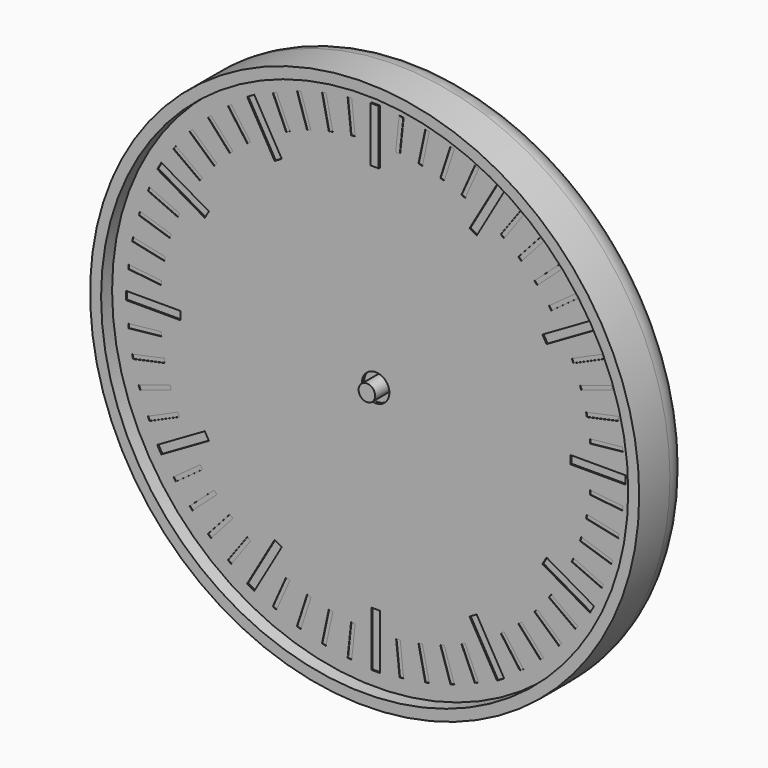
from build123d import *

# Parameters (mm, degrees)
F0_R      = 100
F1_DEPTH  = 24
F2_R      = 10
F3_T      = -4
F4_R      = 5
F4_R_2    = 3
F5_DEPTH  = 2
F6_DEPTH  = 19
F7_DEPTH  = 8
F9_DEPTH  = 4
F11_DEPTH = 4
F12_R     = 5
F12_R_2   = 3
F13_DEPTH = 2
F14_R     = 3
F15_DEPTH = 4
F17_DEPTH = 4
F18_R     = 3
F19_DEPTH = 2
F20_R     = 98
F20_R_2   = 5
F21_DEPTH = 1
F23_R     = 5
F23_R_2   = 3
F24_DEPTH = 2
F25_W     = 3
F25_H     = 20
F25_W_2   = 20
F25_H_2   = 3
F26_DEPTH = 0.5
F27_W     = 1.5
F27_H     = 12
F27_W_2   = 12
F27_H_2   = 1.5
F28_DEPTH = 0.2
F29_DEPTH = 1
F30_DEPTH = 0.4


with BuildPart() as f1:
    # F0 (on Front) → F1 (new body)
    with BuildSketch(Plane.XZ):
        Circle(F0_R)
    extrude(amount=F1_DEPTH)

    # F2
    f2_edges = [f1.edges().sort_by_distance(p)[0] for p in [
        (-100, 0, 0),
    ]]
    fillet(f2_edges, radius=F2_R)

    # F3
    f3_openings = [f1.faces().sort_by_distance(p)[0] for p in [
        (0, -24, 0),
    ]]
    offset(amount=F3_T, openings=f3_openings)

    # F4 (on face) → F5 (join)
    with BuildSketch(Plane.XZ.offset(4)):
        Circle(F4_R)
        Circle(F4_R_2, mode=Mode.SUBTRACT)
        with Locations((40, 0)):
            Circle(F4_R)
        with Locations((40, 0)):
            Circle(F4_R_2, mode=Mode.SUBTRACT)
    extrude(amount=F5_DEPTH)


with BuildPart() as f6:
    # F6 (new): a face of the model
    f6_faces = [f1.part.faces().sort_by_distance(p)[0] for p in [
        (0, -4, 0),
    ]]
    extrude(f6_faces, amount=F6_DEPTH)

    # F8 (on face) → F9 (join)
    with BuildSketch(Plane.XZ.offset(6)):
        with BuildLine():
            ThreePointArc((9.2729637667, -1.3794085621), (9.3494561423, -0.6915886375), (9.375, 0))
            ThreePointArc((9.375, 0), (9.3494561423, 0.6915886375), (9.2729637667, 1.3794085621))
            ThreePointArc((9.2729637667, 1.3794085621), (8.9161548403, 2.8970343223), (8.3127812852, 4.3345463782))
            ThreePointArc((8.3127812852, 4.3345463782), (7.5845343223, 5.5104867402), (6.6911892658, 6.566476316))
            ThreePointArc((6.6911892658, 6.566476316), (5.5104867402, 7.5845343223), (4.1773988938, 8.3928519278))
            ThreePointArc((4.1773988938, 8.3928519278), (2.8970343223, 8.9161548403), (1.5536078905, 9.2453733036))
            ThreePointArc((1.5536078905, 9.2453733036), (0, 9.375), (-1.5536078905, 9.2453733036))
            ThreePointArc((-1.5536078905, 9.2453733036), (-2.8970343223, 8.9161548403), (-4.1773988938, 8.3928519278))
            ThreePointArc((-4.1773988938, 8.3928519278), (-5.5104867402, 7.5845343223), (-6.6911892658, 6.566476316))
            ThreePointArc((-6.6911892658, 6.566476316), (-7.5845343223, 5.5104867402), (-8.3127812852, 4.3345463782))
            ThreePointArc((-8.3127812852, 4.3345463782), (-8.9161548403, 2.8970343223), (-9.2729637667, 1.3794085621))
            ThreePointArc((-9.2729637667, 1.3794085621), (-9.375, 0), (-9.2729637667, -1.3794085621))
            ThreePointArc((-9.2729637667, -1.3794085621), (-8.9161548403, -2.8970343223), (-8.3127812852, -4.3345463782))
            ThreePointArc((-8.3127812852, -4.3345463782), (-7.5845343223, -5.5104867402), (-6.6911892658, -6.566476316))
            ThreePointArc((-6.6911892658, -6.566476316), (-5.5104867402, -7.5845343223), (-4.1773988938, -8.3928519278))
            ThreePointArc((-4.1773988938, -8.3928519278), (-2.8970343223, -8.9161548403), (-1.5536078905, -9.2453733036))
            ThreePointArc((-1.5536078905, -9.2453733036), (0, -9.375), (1.5536078905, -9.2453733036))
            ThreePointArc((1.5536078905, -9.2453733036), (2.8970343223, -8.9161548403), (4.1773988938, -8.3928519278))
            ThreePointArc((4.1773988938, -8.3928519278), (5.5104867402, -7.5845343223), (6.6911892658, -6.566476316))
            ThreePointArc((6.6911892658, -6.566476316), (7.5845343223, -5.5104867402), (8.3127812852, -4.3345463782))
            ThreePointArc((8.3127812852, -4.3345463782), (8.9161548403, -2.8970343223), (9.2729637667, -1.3794085621))
        make_face()
        with BuildLine():
            ThreePointArc((8.3127812852, 4.3345463782), (8.9161548403, 2.8970343223), (9.2729637667, 1.3794085621))
            Line((9.2729637667, 1.3794085621), (11.1823199426, 2.3946312492))
            Line((11.1823199426, 2.3946312492), (10.8182678729, 3.515068311))
            Line((10.8182678729, 3.515068311), (10.4542158031, 4.6355053728))
            Line((10.4542158031, 4.6355053728), (8.3127812852, 4.3345463782))
        make_face()
        with BuildLine():
            Line((11.1823199426, -2.3946312492), (9.2729637667, -1.3794085621))
            ThreePointArc((9.2729637667, -1.3794085621), (8.9161548403, -2.8970343223), (8.3127812852, -4.3345463782))
            Line((8.3127812852, -4.3345463782), (10.4542158031, -4.6355053728))
            Line((10.4542158031, -4.6355053728), (10.8182678729, -3.515068311))
            Line((10.8182678729, -3.515068311), (11.1823199426, -2.3946312492))
        make_face()
        with BuildLine():
            ThreePointArc((4.1773988938, 8.3928519278), (5.5104867402, 7.5845343223), (6.6911892658, 6.566476316))
            Line((6.6911892658, 6.566476316), (7.6391579371, 8.5101001246))
            Line((7.6391579371, 8.5101001246), (6.6860572448, 9.202568311))
            Line((6.6860572448, 9.202568311), (5.7329565525, 9.8950364974))
            Line((5.7329565525, 9.8950364974), (4.1773988938, 8.3928519278))
        make_face()
        with BuildLine():
            Line((7.6391579371, -8.5101001246), (6.6911892658, -6.566476316))
            ThreePointArc((6.6911892658, -6.566476316), (5.5104867402, -7.5845343223), (4.1773988938, -8.3928519278))
            Line((4.1773988938, -8.3928519278), (5.7329565525, -9.8950364974))
            Line((5.7329565525, -9.8950364974), (6.6860572448, -9.202568311))
            Line((6.6860572448, -9.202568311), (7.6391579371, -8.5101001246))
        make_face()
        with BuildLine():
            ThreePointArc((-1.5536078905, 9.2453733036), (0, 9.375), (1.5536078905, 9.2453733036))
            Line((1.5536078905, 9.2453733036), (1.1780972451, 11.375))
            Line((1.1780972451, 11.375), (0, 11.375))
            Line((0, 11.375), (-1.1780972451, 11.375))
            Line((-1.1780972451, 11.375), (-1.5536078905, 9.2453733036))
        make_face()
        with BuildLine():
            Line((1.1780972451, -11.375), (1.5536078905, -9.2453733036))
            ThreePointArc((1.5536078905, -9.2453733036), (0, -9.375), (-1.5536078905, -9.2453733036))
            Line((-1.5536078905, -9.2453733036), (-1.1780972451, -11.375))
            Line((-1.1780972451, -11.375), (0, -11.375))
            Line((0, -11.375), (1.1780972451, -11.375))
        make_face()
        with BuildLine():
            ThreePointArc((-6.6911892658, 6.566476316), (-5.5104867402, 7.5845343223), (-4.1773988938, 8.3928519278))
            Line((-4.1773988938, 8.3928519278), (-5.7329565525, 9.8950364974))
            Line((-5.7329565525, 9.8950364974), (-6.6860572448, 9.202568311))
            Line((-6.6860572448, 9.202568311), (-7.6391579371, 8.5101001246))
            Line((-7.6391579371, 8.5101001246), (-6.6911892658, 6.566476316))
        make_face()
        with BuildLine():
            Line((-5.7329565525, -9.8950364974), (-4.1773988938, -8.3928519278))
            ThreePointArc((-4.1773988938, -8.3928519278), (-5.5104867402, -7.5845343223), (-6.6911892658, -6.566476316))
            Line((-6.6911892658, -6.566476316), (-7.6391579371, -8.5101001246))
            Line((-7.6391579371, -8.5101001246), (-6.6860572448, -9.202568311))
            Line((-6.6860572448, -9.202568311), (-5.7329565525, -9.8950364974))
        make_face()
        with BuildLine():
            ThreePointArc((-9.2729637667, 1.3794085621), (-8.9161548403, 2.8970343223), (-8.3127812852, 4.3345463782))
            Line((-8.3127812852, 4.3345463782), (-10.4542158031, 4.6355053728))
            Line((-10.4542158031, 4.6355053728), (-10.8182678729, 3.515068311))
            Line((-10.8182678729, 3.515068311), (-11.1823199426, 2.3946312492))
            Line((-11.1823199426, 2.3946312492), (-9.2729637667, 1.3794085621))
        make_face()
        with BuildLine():
            Line((-10.4542158031, -4.6355053728), (-8.3127812852, -4.3345463782))
            ThreePointArc((-8.3127812852, -4.3345463782), (-8.9161548403, -2.8970343223), (-9.2729637667, -1.3794085621))
            Line((-9.2729637667, -1.3794085621), (-11.1823199426, -2.3946312492))
            Line((-11.1823199426, -2.3946312492), (-10.8182678729, -3.515068311))
            Line((-10.8182678729, -3.515068311), (-10.4542158031, -4.6355053728))
        make_face()
    extrude(amount=F9_DEPTH)


with BuildPart() as f7:
    # F7 (new): a face of the model
    f7_faces = [f1.part.faces().sort_by_distance(p)[0] for p in [
        (40, -4, 0),
    ]]
    extrude(f7_faces, amount=F7_DEPTH)

    # F10 (on face) → F11 (join)
    with BuildSketch(Plane.XZ.offset(6)):
        with BuildLine():
            ThreePointArc((68.0829066802, -1.5381733945), (68.1144747006, -0.7693746225), (68.125, 0))
            ThreePointArc((68.125, 0), (68.1144747006, 0.7693746225), (68.0829066802, 1.5381733945))
            ThreePointArc((68.0829066802, 1.5381733945), (67.9709283072, 2.9398630294), (67.7890320221, 4.3342039956))
            ThreePointArc((67.7890320221, 4.3342039956), (67.5104012706, 5.8475163042), (67.1494235596, 7.3433252263))
            ThreePointArc((67.1494235596, 7.3433252263), (66.7484645208, 8.6911029668), (66.280643318, 10.0171558733))
            ThreePointArc((66.280643318, 10.0171558733), (65.6934659962, 11.4394680865), (65.0293803521, 12.8275385085))
            ThreePointArc((65.0293803521, 12.8275385085), (64.3569644814, 14.0625), (63.6236643925, 15.2623099717))
            ThreePointArc((63.6236643925, 15.2623099717), (62.7536029668, 16.5314602207), (61.815433119, 17.7511268046))
            ThreePointArc((61.815433119, 17.7511268046), (60.9009482166, 18.8192983038), (59.934217974, 19.8404278876))
            ThreePointArc((59.934217974, 19.8404278876), (58.8192983038, 20.9009482166), (57.6480467764, 21.8989056799))
            ThreePointArc((57.6480467764, 21.8989056799), (56.5314602207, 22.7536029668), (55.3735505752, 23.5514238999))
            ThreePointArc((55.3735505752, 23.5514238999), (54.0625, 24.3569644814), (52.709356105, 25.0895972944))
            ThreePointArc((52.709356105, 25.0895972944), (51.4394680865, 25.6934659962), (50.1409852457, 26.2331096755))
            ThreePointArc((50.1409852457, 26.2331096755), (48.6911029668, 26.7484645208), (47.2152055856, 27.1837531139))
            ThreePointArc((47.2152055856, 27.1837531139), (45.8475163042, 27.5104012706), (44.4652101991, 27.7682826779))
            ThreePointArc((44.4652101991, 27.7682826779), (42.9398630294, 27.9709283072), (41.4057159597, 28.0898484802))
            ThreePointArc((41.4057159597, 28.0898484802), (40, 28.125), (38.5942840403, 28.0898484802))
            ThreePointArc((38.5942840403, 28.0898484802), (37.0601369706, 27.9709283072), (35.5347898009, 27.7682826779))
            ThreePointArc((35.5347898009, 27.7682826779), (34.1524836958, 27.5104012706), (32.7847944144, 27.1837531139))
            ThreePointArc((32.7847944144, 27.1837531139), (31.3088970332, 26.7484645208), (29.8590147543, 26.2331096755))
            ThreePointArc((29.8590147543, 26.2331096755), (28.5605319135, 25.6934659962), (27.290643895, 25.0895972944))
            ThreePointArc((27.290643895, 25.0895972944), (25.9375, 24.3569644814), (24.6264494248, 23.5514238999))
            ThreePointArc((24.6264494248, 23.5514238999), (23.4685397793, 22.7536029668), (22.3519532236, 21.8989056799))
            ThreePointArc((22.3519532236, 21.8989056799), (21.1807016962, 20.9009482166), (20.065782026, 19.8404278876))
            ThreePointArc((20.065782026, 19.8404278876), (19.0990517834, 18.8192983038), (18.184566881, 17.7511268046))
            ThreePointArc((18.184566881, 17.7511268046), (17.2463970332, 16.5314602207), (16.3763356075, 15.2623099717))
            ThreePointArc((16.3763356075, 15.2623099717), (15.6430355186, 14.0625), (14.9706196479, 12.8275385085))
            ThreePointArc((14.9706196479, 12.8275385085), (14.3065340038, 11.4394680865), (13.719356682, 10.0171558733))
            ThreePointArc((13.719356682, 10.0171558733), (13.2515354792, 8.6911029668), (12.8505764404, 7.3433252263))
            ThreePointArc((12.8505764404, 7.3433252263), (12.4895987294, 5.8475163042), (12.2109679779, 4.3342039956))
            ThreePointArc((12.2109679779, 4.3342039956), (12.0290716928, 2.9398630294), (11.9170933198, 1.5381733945))
            ThreePointArc((11.9170933198, 1.5381733945), (11.875, 0), (11.9170933198, -1.5381733945))
            ThreePointArc((11.9170933198, -1.5381733945), (12.0290716928, -2.9398630294), (12.2109679779, -4.3342039956))
            ThreePointArc((12.2109679779, -4.3342039956), (12.4895987294, -5.8475163042), (12.8505764404, -7.3433252263))
            ThreePointArc((12.8505764404, -7.3433252263), (13.2515354792, -8.6911029668), (13.719356682, -10.0171558733))
            ThreePointArc((13.719356682, -10.0171558733), (14.3065340038, -11.4394680865), (14.9706196479, -12.8275385085))
            ThreePointArc((14.9706196479, -12.8275385085), (15.6430355186, -14.0625), (16.3763356075, -15.2623099717))
            ThreePointArc((16.3763356075, -15.2623099717), (17.2463970332, -16.5314602207), (18.184566881, -17.7511268046))
            ThreePointArc((18.184566881, -17.7511268046), (19.0990517834, -18.8192983038), (20.065782026, -19.8404278876))
            ThreePointArc((20.065782026, -19.8404278876), (21.1807016962, -20.9009482166), (22.3519532236, -21.8989056799))
            ThreePointArc((22.3519532236, -21.8989056799), (23.4685397793, -22.7536029668), (24.6264494248, -23.5514238999))
            ThreePointArc((24.6264494248, -23.5514238999), (25.9375, -24.3569644814), (27.290643895, -25.0895972944))
            ThreePointArc((27.290643895, -25.0895972944), (28.5605319135, -25.6934659962), (29.8590147543, -26.2331096755))
            ThreePointArc((29.8590147543, -26.2331096755), (31.3088970332, -26.7484645208), (32.7847944144, -27.1837531139))
            ThreePointArc((32.7847944144, -27.1837531139), (34.1524836958, -27.5104012706), (35.5347898009, -27.7682826779))
            ThreePointArc((35.5347898009, -27.7682826779), (37.0601369706, -27.9709283072), (38.5942840403, -28.0898484802))
            ThreePointArc((38.5942840403, -28.0898484802), (40, -28.125), (41.4057159597, -28.0898484802))
            ThreePointArc((41.4057159597, -28.0898484802), (42.9398630294, -27.9709283072), (44.4652101991, -27.7682826779))
            ThreePointArc((44.4652101991, -27.7682826779), (45.8475163042, -27.5104012706), (47.2152055856, -27.1837531139))
            ThreePointArc((47.2152055856, -27.1837531139), (48.6911029668, -26.7484645208), (50.1409852457, -26.2331096755))
            ThreePointArc((50.1409852457, -26.2331096755), (51.4394680865, -25.6934659962), (52.709356105, -25.0895972944))
            ThreePointArc((52.709356105, -25.0895972944), (54.0625, -24.3569644814), (55.3735505752, -23.5514238999))
            ThreePointArc((55.3735505752, -23.5514238999), (56.5314602207, -22.7536029668), (57.6480467764, -21.8989056799))
            ThreePointArc((57.6480467764, -21.8989056799), (58.8192983038, -20.9009482166), (59.934217974, -19.8404278876))
            ThreePointArc((59.934217974, -19.8404278876), (60.9009482166, -18.8192983038), (61.815433119, -17.7511268046))
            ThreePointArc((61.815433119, -17.7511268046), (62.7536029668, -16.5314602207), (63.6236643925, -15.2623099717))
            ThreePointArc((63.6236643925, -15.2623099717), (64.3569644814, -14.0625), (65.0293803521, -12.8275385085))
            ThreePointArc((65.0293803521, -12.8275385085), (65.6934659962, -11.4394680865), (66.280643318, -10.0171558733))
            ThreePointArc((66.280643318, -10.0171558733), (66.7484645208, -8.6911029668), (67.1494235596, -7.3433252263))
            ThreePointArc((67.1494235596, -7.3433252263), (67.5104012706, -5.8475163042), (67.7890320221, -4.3342039956))
            ThreePointArc((67.7890320221, -4.3342039956), (67.9709283072, -2.9398630294), (68.0829066802, -1.5381733945))
        make_face()
        with BuildLine():
            ThreePointArc((68.0829066802, 1.5381733945), (68.1144747006, 0.7693746225), (68.125, 0))
            ThreePointArc((68.125, 0), (68.1144747006, -0.7693746225), (68.0829066802, -1.5381733945))
            Line((68.0829066802, -1.5381733945), (70.125, -1.1780972451))
            Line((70.125, -1.1780972451), (70.125, 0))
            Line((70.125, 0), (70.125, 1.1780972451))
            Line((70.125, 1.1780972451), (68.0829066802, 1.5381733945))
        make_face()
        with BuildLine():
            ThreePointArc((67.1494235596, 7.3433252263), (67.5104012706, 5.8475163042), (67.7890320221, 4.3342039956))
            Line((67.7890320221, 4.3342039956), (69.7116366623, 5.1109866922))
            Line((69.7116366623, 5.1109866922), (69.4666964721, 6.2633396859))
            Line((69.4666964721, 6.2633396859), (69.2217562819, 7.4156926796))
            Line((69.2217562819, 7.4156926796), (67.1494235596, 7.3433252263))
        make_face()
        with BuildLine():
            Line((69.7116366623, -5.1109866922), (67.7890320221, -4.3342039956))
            ThreePointArc((67.7890320221, -4.3342039956), (67.5104012706, -5.8475163042), (67.1494235596, -7.3433252263))
            Line((67.1494235596, -7.3433252263), (69.2217562819, -7.4156926796))
            Line((69.2217562819, -7.4156926796), (69.4666964721, -6.2633396859))
            Line((69.4666964721, -6.2633396859), (69.7116366623, -5.1109866922))
        make_face()
        with BuildLine():
            ThreePointArc((65.0293803521, 12.8275385085), (65.6934659962, 11.4394680865), (66.280643318, 10.0171558733))
            Line((66.280643318, 10.0171558733), (67.9997322302, 11.1766959857))
            Line((67.9997322302, 11.1766959857), (67.5205569115, 12.2529413727))
            Line((67.5205569115, 12.2529413727), (67.0413815928, 13.3291867596))
            Line((67.0413815928, 13.3291867596), (65.0293803521, 12.8275385085))
        make_face()
        with BuildLine():
            Line((67.9997322302, -11.1766959857), (66.280643318, -10.0171558733))
            ThreePointArc((66.280643318, -10.0171558733), (65.6934659962, -11.4394680865), (65.0293803521, -12.8275385085))
            Line((65.0293803521, -12.8275385085), (67.0413815928, -13.3291867596))
            Line((67.0413815928, -13.3291867596), (67.5205569115, -12.2529413727))
            Line((67.5205569115, -12.2529413727), (67.9997322302, -11.1766959857))
        make_face()
        with BuildLine():
            ThreePointArc((61.815433119, 17.7511268046), (62.7536029668, 16.5314602207), (63.6236643925, 15.2623099717))
            Line((63.6236643925, 15.2623099717), (65.064105142, 16.753930033))
            Line((65.064105142, 16.753930033), (64.3716369555, 17.7070307253))
            Line((64.3716369555, 17.7070307253), (63.6791687691, 18.6601314176))
            Line((63.6791687691, 18.6601314176), (61.815433119, 17.7511268046))
        make_face()
        with BuildLine():
            Line((65.064105142, -16.753930033), (63.6236643925, -15.2623099717))
            ThreePointArc((63.6236643925, -15.2623099717), (62.7536029668, -16.5314602207), (61.815433119, -17.7511268046))
            Line((61.815433119, -17.7511268046), (63.6791687691, -18.6601314176))
            Line((63.6791687691, -18.6601314176), (64.3716369555, -17.7070307253))
            Line((64.3716369555, -17.7070307253), (65.064105142, -16.753930033))
        make_face()
        with BuildLine():
            ThreePointArc((57.6480467764, 21.8989056799), (58.8192983038, 20.9009482166), (59.934217974, 19.8404278876))
            Line((59.934217974, 19.8404278876), (61.0330563882, 21.5989369435))
            Line((61.0330563882, 21.5989369435), (60.1575595166, 22.3872378675))
            Line((60.1575595166, 22.3872378675), (59.282062645, 23.1755387915))
            Line((59.282062645, 23.1755387915), (57.6480467764, 21.8989056799))
        make_face()
        with BuildLine():
            Line((61.0330563882, -21.5989369435), (59.934217974, -19.8404278876))
            ThreePointArc((59.934217974, -19.8404278876), (58.8192983038, -20.9009482166), (57.6480467764, -21.8989056799))
            Line((57.6480467764, -21.8989056799), (59.282062645, -23.1755387915))
            Line((59.282062645, -23.1755387915), (60.1575595166, -22.3872378675))
            Line((60.1575595166, -22.3872378675), (61.0330563882, -21.5989369435))
        make_face()
        with BuildLine():
            ThreePointArc((52.709356105, 25.0895972944), (54.0625, 24.3569644814), (55.3735505752, 23.5514238999))
            Line((55.3735505752, 23.5514238999), (56.0827621424, 25.4999666665))
            Line((56.0827621424, 25.4999666665), (55.0625, 26.089015289))
            Line((55.0625, 26.089015289), (54.0422378576, 26.6780639116))
            Line((54.0422378576, 26.6780639116), (52.709356105, 25.0895972944))
        make_face()
        with BuildLine():
            Line((56.0827621424, -25.4999666665), (55.3735505752, -23.5514238999))
            ThreePointArc((55.3735505752, -23.5514238999), (54.0625, -24.3569644814), (52.709356105, -25.0895972944))
            Line((52.709356105, -25.0895972944), (54.0422378576, -26.6780639116))
            Line((54.0422378576, -26.6780639116), (55.0625, -26.089015289))
            Line((55.0625, -26.089015289), (56.0827621424, -25.4999666665))
        make_face()
        with BuildLine():
            ThreePointArc((47.2152055856, 27.1837531139), (48.6911029668, 26.7484645208), (50.1409852457, 26.2331096755))
            Line((50.1409852457, 26.2331096755), (50.4295740173, 28.2865254836))
            Line((50.4295740173, 28.2865254836), (49.3091369555, 28.6505775534))
            Line((49.3091369555, 28.6505775534), (48.1886998938, 29.0146296232))
            Line((48.1886998938, 29.0146296232), (47.2152055856, 27.1837531139))
        make_face()
        with BuildLine():
            Line((50.4295740173, -28.2865254836), (50.1409852457, -26.2331096755))
            ThreePointArc((50.1409852457, -26.2331096755), (48.6911029668, -26.7484645208), (47.2152055856, -27.1837531139))
            Line((47.2152055856, -27.1837531139), (48.1886998938, -29.0146296232))
            Line((48.1886998938, -29.0146296232), (49.3091369555, -28.6505775534))
            Line((49.3091369555, -28.6505775534), (50.4295740173, -28.2865254836))
        make_face()
        with BuildLine():
            ThreePointArc((41.4057159597, 28.0898484802), (42.9398630294, 27.9709283072), (44.4652101991, 27.7682826779))
            Line((44.4652101991, 27.7682826779), (44.3205634611, 29.8368274034))
            Line((44.3205634611, 29.8368274034), (43.1489199559, 29.959972098))
            Line((43.1489199559, 29.959972098), (41.9772764508, 30.0831167926))
            Line((41.9772764508, 30.0831167926), (41.4057159597, 28.0898484802))
        make_face()
        with BuildLine():
            Line((44.3205634611, -29.8368274034), (44.4652101991, -27.7682826779))
            ThreePointArc((44.4652101991, -27.7682826779), (42.9398630294, -27.9709283072), (41.4057159597, -28.0898484802))
            Line((41.4057159597, -28.0898484802), (41.9772764508, -30.0831167926))
            Line((41.9772764508, -30.0831167926), (43.1489199559, -29.959972098))
            Line((43.1489199559, -29.959972098), (44.3205634611, -29.8368274034))
        make_face()
        with BuildLine():
            ThreePointArc((35.5347898009, 27.7682826779), (37.0601369706, 27.9709283072), (38.5942840403, 28.0898484802))
            Line((38.5942840403, 28.0898484802), (38.0227235492, 30.0831167926))
            Line((38.0227235492, 30.0831167926), (36.8510800441, 29.959972098))
            Line((36.8510800441, 29.959972098), (35.6794365389, 29.8368274034))
            Line((35.6794365389, 29.8368274034), (35.5347898009, 27.7682826779))
        make_face()
        with BuildLine():
            Line((38.0227235492, -30.0831167926), (38.5942840403, -28.0898484802))
            ThreePointArc((38.5942840403, -28.0898484802), (37.0601369706, -27.9709283072), (35.5347898009, -27.7682826779))
            Line((35.5347898009, -27.7682826779), (35.6794365389, -29.8368274034))
            Line((35.6794365389, -29.8368274034), (36.8510800441, -29.959972098))
            Line((36.8510800441, -29.959972098), (38.0227235492, -30.0831167926))
        make_face()
        with BuildLine():
            ThreePointArc((29.8590147543, 26.2331096755), (31.3088970332, 26.7484645208), (32.7847944144, 27.1837531139))
            Line((32.7847944144, 27.1837531139), (31.8113001062, 29.0146296232))
            Line((31.8113001062, 29.0146296232), (30.6908630445, 28.6505775534))
            Line((30.6908630445, 28.6505775534), (29.5704259827, 28.2865254836))
            Line((29.5704259827, 28.2865254836), (29.8590147543, 26.2331096755))
        make_face()
        with BuildLine():
            Line((31.8113001062, -29.0146296232), (32.7847944144, -27.1837531139))
            ThreePointArc((32.7847944144, -27.1837531139), (31.3088970332, -26.7484645208), (29.8590147543, -26.2331096755))
            Line((29.8590147543, -26.2331096755), (29.5704259827, -28.2865254836))
            Line((29.5704259827, -28.2865254836), (30.6908630445, -28.6505775534))
            Line((30.6908630445, -28.6505775534), (31.8113001062, -29.0146296232))
        make_face()
        with BuildLine():
            ThreePointArc((24.6264494248, 23.5514238999), (25.9375, 24.3569644814), (27.290643895, 25.0895972944))
            Line((27.290643895, 25.0895972944), (25.9577621424, 26.6780639116))
            Line((25.9577621424, 26.6780639116), (24.9375, 26.089015289))
            Line((24.9375, 26.089015289), (23.9172378576, 25.4999666665))
            Line((23.9172378576, 25.4999666665), (24.6264494248, 23.5514238999))
        make_face()
        with BuildLine():
            Line((25.9577621424, -26.6780639116), (27.290643895, -25.0895972944))
            ThreePointArc((27.290643895, -25.0895972944), (25.9375, -24.3569644814), (24.6264494248, -23.5514238999))
            Line((24.6264494248, -23.5514238999), (23.9172378576, -25.4999666665))
            Line((23.9172378576, -25.4999666665), (24.9375, -26.089015289))
            Line((24.9375, -26.089015289), (25.9577621424, -26.6780639116))
        make_face()
        with BuildLine():
            ThreePointArc((20.065782026, 19.8404278876), (21.1807016962, 20.9009482166), (22.3519532236, 21.8989056799))
            Line((22.3519532236, 21.8989056799), (20.717937355, 23.1755387915))
            Line((20.717937355, 23.1755387915), (19.8424404834, 22.3872378675))
            Line((19.8424404834, 22.3872378675), (18.9669436118, 21.5989369435))
            Line((18.9669436118, 21.5989369435), (20.065782026, 19.8404278876))
        make_face()
        with BuildLine():
            Line((20.717937355, -23.1755387915), (22.3519532236, -21.8989056799))
            ThreePointArc((22.3519532236, -21.8989056799), (21.1807016962, -20.9009482166), (20.065782026, -19.8404278876))
            Line((20.065782026, -19.8404278876), (18.9669436118, -21.5989369435))
            Line((18.9669436118, -21.5989369435), (19.8424404834, -22.3872378675))
            Line((19.8424404834, -22.3872378675), (20.717937355, -23.1755387915))
        make_face()
        with BuildLine():
            ThreePointArc((16.3763356075, 15.2623099717), (17.2463970332, 16.5314602207), (18.184566881, 17.7511268046))
            Line((18.184566881, 17.7511268046), (16.3208312309, 18.6601314176))
            Line((16.3208312309, 18.6601314176), (15.6283630445, 17.7070307253))
            Line((15.6283630445, 17.7070307253), (14.935894858, 16.753930033))
            Line((14.935894858, 16.753930033), (16.3763356075, 15.2623099717))
        make_face()
        with BuildLine():
            Line((16.3208312309, -18.6601314176), (18.184566881, -17.7511268046))
            ThreePointArc((18.184566881, -17.7511268046), (17.2463970332, -16.5314602207), (16.3763356075, -15.2623099717))
            Line((16.3763356075, -15.2623099717), (14.935894858, -16.753930033))
            Line((14.935894858, -16.753930033), (15.6283630445, -17.7070307253))
            Line((15.6283630445, -17.7070307253), (16.3208312309, -18.6601314176))
        make_face()
        with BuildLine():
            ThreePointArc((13.719356682, 10.0171558733), (14.3065340038, 11.4394680865), (14.9706196479, 12.8275385085))
            Line((14.9706196479, 12.8275385085), (12.9586184072, 13.3291867596))
            Line((12.9586184072, 13.3291867596), (12.4794430885, 12.2529413727))
            Line((12.4794430885, 12.2529413727), (12.0002677698, 11.1766959857))
            Line((12.0002677698, 11.1766959857), (13.719356682, 10.0171558733))
        make_face()
        with BuildLine():
            Line((12.9586184072, -13.3291867596), (14.9706196479, -12.8275385085))
            ThreePointArc((14.9706196479, -12.8275385085), (14.3065340038, -11.4394680865), (13.719356682, -10.0171558733))
            Line((13.719356682, -10.0171558733), (12.0002677698, -11.1766959857))
            Line((12.0002677698, -11.1766959857), (12.4794430885, -12.2529413727))
            Line((12.4794430885, -12.2529413727), (12.9586184072, -13.3291867596))
        make_face()
        with BuildLine():
            ThreePointArc((12.2109679779, 4.3342039956), (12.4895987294, 5.8475163042), (12.8505764404, 7.3433252263))
            Line((12.8505764404, 7.3433252263), (10.7782437181, 7.4156926796))
            Line((10.7782437181, 7.4156926796), (10.5333035279, 6.2633396859))
            Line((10.5333035279, 6.2633396859), (10.2883633377, 5.1109866922))
            Line((10.2883633377, 5.1109866922), (12.2109679779, 4.3342039956))
        make_face()
        with BuildLine():
            Line((10.7782437181, -7.4156926796), (12.8505764404, -7.3433252263))
            ThreePointArc((12.8505764404, -7.3433252263), (12.4895987294, -5.8475163042), (12.2109679779, -4.3342039956))
            Line((12.2109679779, -4.3342039956), (10.2883633377, -5.1109866922))
            Line((10.2883633377, -5.1109866922), (10.5333035279, -6.2633396859))
            Line((10.5333035279, -6.2633396859), (10.7782437181, -7.4156926796))
        make_face()
        with BuildLine():
            ThreePointArc((11.9170933198, -1.5381733945), (11.875, 0), (11.9170933198, 1.5381733945))
            Line((11.9170933198, 1.5381733945), (9.875, 1.1780972451))
            Line((9.875, 1.1780972451), (9.875, 0))
            Line((9.875, 0), (9.875, -1.1780972451))
            Line((9.875, -1.1780972451), (11.9170933198, -1.5381733945))
        make_face()
    extrude(amount=F11_DEPTH)

    # F16 (on face) → F17 (join)
    with BuildSketch(Plane.XZ.offset(12)):
        with BuildLine():
            ThreePointArc((47.4288750323, -1.0304444454), (47.4821976298, -0.5164480894), (47.5, 0))
            ThreePointArc((47.5, 0), (47.4821976298, 0.5164480894), (47.4288750323, 1.0304444454))
            ThreePointArc((47.4288750323, 1.0304444454), (47.1329238722, 2.3176274578), (46.6157661985, 3.532936117))
            ThreePointArc((46.6157661985, 3.532936117), (46.0676274578, 4.4083893922), (45.4044061018, 5.2002302532))
            ThreePointArc((45.4044061018, 5.2002302532), (44.4083893922, 6.0676274578), (43.2756595386, 6.7468551628))
            ThreePointArc((43.2756595386, 6.7468551628), (42.3176274578, 7.1329238722), (41.3156377295, 7.3837048536))
            ThreePointArc((41.3156377295, 7.3837048536), (40, 7.5), (38.6843622705, 7.3837048536))
            ThreePointArc((38.6843622705, 7.3837048536), (37.6823725422, 7.1329238722), (36.7243404614, 6.7468551628))
            ThreePointArc((36.7243404614, 6.7468551628), (35.5916106078, 6.0676274578), (34.5955938982, 5.2002302532))
            ThreePointArc((34.5955938982, 5.2002302532), (33.9323725422, 4.4083893922), (33.3842338015, 3.532936117))
            ThreePointArc((33.3842338015, 3.532936117), (32.8670761278, 2.3176274578), (32.5711249677, 1.0304444454))
            ThreePointArc((32.5711249677, 1.0304444454), (32.5, 0), (32.5711249677, -1.0304444454))
            ThreePointArc((32.5711249677, -1.0304444454), (32.8670761278, -2.3176274578), (33.3842338015, -3.532936117))
            ThreePointArc((33.3842338015, -3.532936117), (33.9323725422, -4.4083893922), (34.5955938982, -5.2002302532))
            ThreePointArc((34.5955938982, -5.2002302532), (35.5916106078, -6.0676274578), (36.7243404614, -6.7468551628))
            ThreePointArc((36.7243404614, -6.7468551628), (37.6823725422, -7.1329238722), (38.6843622705, -7.3837048536))
            ThreePointArc((38.6843622705, -7.3837048536), (40, -7.5), (41.3156377295, -7.3837048536))
            ThreePointArc((41.3156377295, -7.3837048536), (42.3176274578, -7.1329238722), (43.2756595386, -6.7468551628))
            ThreePointArc((43.2756595386, -6.7468551628), (44.4083893922, -6.0676274578), (45.4044061018, -5.2002302532))
            ThreePointArc((45.4044061018, -5.2002302532), (46.0676274578, -4.4083893922), (46.6157661985, -3.532936117))
            ThreePointArc((46.6157661985, -3.532936117), (47.1329238722, -2.3176274578), (47.4288750323, -1.0304444454))
        make_face()
        with BuildLine():
            ThreePointArc((46.6157661985, 3.532936117), (47.1329238722, 2.3176274578), (47.4288750323, 1.0304444454))
            Line((47.4288750323, 1.0304444454), (49.3262785606, 2.0393117971))
            Line((49.3262785606, 2.0393117971), (48.743795249, 3.832011096))
            Line((48.743795249, 3.832011096), (46.6157661985, 3.532936117))
        make_face()
        with BuildLine():
            Line((49.3262785606, -2.0393117971), (47.4288750323, -1.0304444454))
            ThreePointArc((47.4288750323, -1.0304444454), (47.1329238722, -2.3176274578), (46.6157661985, -3.532936117))
            Line((46.6157661985, -3.532936117), (48.743795249, -3.832011096))
            Line((48.743795249, -3.832011096), (49.3262785606, -2.0393117971))
        make_face()
        with BuildLine():
            ThreePointArc((43.2756595386, 6.7468551628), (44.4083893922, 6.0676274578), (45.4044061018, 5.2002302532))
            Line((45.4044061018, 5.2002302532), (46.3464404506, 7.1316868974))
            Line((46.3464404506, 7.1316868974), (44.8214793429, 8.2396359957))
            Line((44.8214793429, 8.2396359957), (43.2756595386, 6.7468551628))
        make_face()
        with BuildLine():
            Line((46.3464404506, -7.1316868974), (45.4044061018, -5.2002302532))
            ThreePointArc((45.4044061018, -5.2002302532), (44.4083893922, -6.0676274578), (43.2756595386, -6.7468551628))
            Line((43.2756595386, -6.7468551628), (44.8214793429, -8.2396359957))
            Line((44.8214793429, -8.2396359957), (46.3464404506, -7.1316868974))
        make_face()
        with BuildLine():
            ThreePointArc((38.6843622705, 7.3837048536), (40, 7.5), (41.3156377295, 7.3837048536))
            Line((41.3156377295, 7.3837048536), (40.9424777961, 9.5))
            Line((40.9424777961, 9.5), (39.0575222039, 9.5))
            Line((39.0575222039, 9.5), (38.6843622705, 7.3837048536))
        make_face()
        with BuildLine():
            Line((40.9424777961, -9.5), (41.3156377295, -7.3837048536))
            ThreePointArc((41.3156377295, -7.3837048536), (40, -7.5), (38.6843622705, -7.3837048536))
            Line((38.6843622705, -7.3837048536), (39.0575222039, -9.5))
            Line((39.0575222039, -9.5), (40.9424777961, -9.5))
        make_face()
        with BuildLine():
            ThreePointArc((34.5955938982, 5.2002302532), (35.5916106078, 6.0676274578), (36.7243404614, 6.7468551628))
            Line((36.7243404614, 6.7468551628), (35.1785206571, 8.2396359957))
            Line((35.1785206571, 8.2396359957), (33.6535595494, 7.1316868974))
            Line((33.6535595494, 7.1316868974), (34.5955938982, 5.2002302532))
        make_face()
        with BuildLine():
            Line((35.1785206571, -8.2396359957), (36.7243404614, -6.7468551628))
            ThreePointArc((36.7243404614, -6.7468551628), (35.5916106078, -6.0676274578), (34.5955938982, -5.2002302532))
            Line((34.5955938982, -5.2002302532), (33.6535595494, -7.1316868974))
            Line((33.6535595494, -7.1316868974), (35.1785206571, -8.2396359957))
        make_face()
        with BuildLine():
            ThreePointArc((32.5711249677, 1.0304444454), (32.8670761278, 2.3176274578), (33.3842338015, 3.532936117))
            Line((33.3842338015, 3.532936117), (31.256204751, 3.832011096))
            Line((31.256204751, 3.832011096), (30.6737214394, 2.0393117971))
            Line((30.6737214394, 2.0393117971), (32.5711249677, 1.0304444454))
        make_face()
        with BuildLine():
            Line((31.256204751, -3.832011096), (33.3842338015, -3.532936117))
            ThreePointArc((33.3842338015, -3.532936117), (32.8670761278, -2.3176274578), (32.5711249677, -1.0304444454))
            Line((32.5711249677, -1.0304444454), (30.6737214394, -2.0393117971))
            Line((30.6737214394, -2.0393117971), (31.256204751, -3.832011096))
        make_face()
    extrude(amount=F17_DEPTH)

    # F18 (on face) → F19 (join)
    with BuildSketch(Plane.XZ.offset(16)):
        with Locations((40, 0)):
            Circle(F18_R)
    extrude(amount=F19_DEPTH)


with BuildPart() as f13:
    # F12 (on face) → F13 (new body)
    with BuildSketch(Plane.XZ.offset(10)):
        Circle(F12_R)
        Circle(F12_R_2, mode=Mode.SUBTRACT)
    extrude(amount=F13_DEPTH)

    # F14 (on face) → F15 (join)
    with BuildSketch(Plane.XZ.offset(12)):
        with BuildLine():
            ThreePointArc((29.9718156995, -1.3001014101), (29.9929530972, -0.6502034357), (30, 0))
            ThreePointArc((30, 0), (29.9929530972, 0.6502034357), (29.9718156995, 1.3001014101))
            ThreePointArc((29.9718156995, 1.3001014101), (29.907520012, 2.3537728718), (29.8061935814, 3.4045299509))
            ThreePointArc((29.8061935814, 3.4045299509), (29.6306502179, 4.6930339512), (29.3994322443, 5.9727199596))
            ThreePointArc((29.3994322443, 5.9727199596), (29.1710976119, 7.0033609157), (28.9066440563, 8.0253304855))
            ThreePointArc((28.9066440563, 8.0253304855), (28.5316954889, 9.2705098312), (28.1031371961, 10.4982703213))
            ThreePointArc((28.1031371961, 10.4982703213), (27.7163859753, 11.480502971), (27.2953170189, 12.448520749))
            ThreePointArc((27.2953170189, 12.448520749), (26.7301957257, 13.6197149922), (26.1148496411, 14.765318426))
            ThreePointArc((26.1148496411, 14.765318426), (25.5792049306, 15.6749569415), (25.0118886885, 16.5651871174))
            ThreePointArc((25.0118886885, 16.5651871174), (24.2705098312, 17.6335575688), (23.4835278178, 18.6687953878))
            ThreePointArc((23.4835278178, 18.6687953878), (22.812178968, 19.4834414499), (22.1125846489, 20.2739636023))
            ThreePointArc((22.1125846489, 20.2739636023), (21.2132034356, 21.2132034356), (20.2739636023, 22.1125846489))
            ThreePointArc((20.2739636023, 22.1125846489), (19.4834414499, 22.812178968), (18.6687953878, 23.4835278178))
            ThreePointArc((18.6687953878, 23.4835278178), (17.6335575688, 24.2705098312), (16.5651871174, 25.0118886885))
            ThreePointArc((16.5651871174, 25.0118886885), (15.6749569415, 25.5792049306), (14.765318426, 26.1148496411))
            ThreePointArc((14.765318426, 26.1148496411), (13.6197149922, 26.7301957257), (12.448520749, 27.2953170189))
            ThreePointArc((12.448520749, 27.2953170189), (11.480502971, 27.7163859753), (10.4982703213, 28.1031371961))
            ThreePointArc((10.4982703213, 28.1031371961), (9.2705098312, 28.5316954889), (8.0253304855, 28.9066440563))
            ThreePointArc((8.0253304855, 28.9066440563), (7.0033609157, 29.1710976119), (5.9727199596, 29.3994322443))
            ThreePointArc((5.9727199596, 29.3994322443), (4.6930339512, 29.6306502179), (3.4045299509, 29.8061935814))
            ThreePointArc((3.4045299509, 29.8061935814), (2.3537728718, 29.907520012), (1.3001014101, 29.9718156995))
            ThreePointArc((1.3001014101, 29.9718156995), (0, 30), (-1.3001014101, 29.9718156995))
            ThreePointArc((-1.3001014101, 29.9718156995), (-2.3537728718, 29.907520012), (-3.4045299509, 29.8061935814))
            ThreePointArc((-3.4045299509, 29.8061935814), (-4.6930339512, 29.6306502179), (-5.9727199596, 29.3994322443))
            ThreePointArc((-5.9727199596, 29.3994322443), (-7.0033609157, 29.1710976119), (-8.0253304855, 28.9066440563))
            ThreePointArc((-8.0253304855, 28.9066440563), (-9.2705098312, 28.5316954889), (-10.4982703213, 28.1031371961))
            ThreePointArc((-10.4982703213, 28.1031371961), (-11.480502971, 27.7163859753), (-12.448520749, 27.2953170189))
            ThreePointArc((-12.448520749, 27.2953170189), (-13.6197149922, 26.7301957257), (-14.765318426, 26.1148496411))
            ThreePointArc((-14.765318426, 26.1148496411), (-15.6749569415, 25.5792049306), (-16.5651871174, 25.0118886885))
            ThreePointArc((-16.5651871174, 25.0118886885), (-17.6335575688, 24.2705098312), (-18.6687953878, 23.4835278178))
            ThreePointArc((-18.6687953878, 23.4835278178), (-19.4834414499, 22.812178968), (-20.2739636023, 22.1125846489))
            ThreePointArc((-20.2739636023, 22.1125846489), (-21.2132034356, 21.2132034356), (-22.1125846489, 20.2739636023))
            ThreePointArc((-22.1125846489, 20.2739636023), (-22.812178968, 19.4834414499), (-23.4835278178, 18.6687953878))
            ThreePointArc((-23.4835278178, 18.6687953878), (-24.2705098312, 17.6335575688), (-25.0118886885, 16.5651871174))
            ThreePointArc((-25.0118886885, 16.5651871174), (-25.5792049306, 15.6749569415), (-26.1148496411, 14.765318426))
            ThreePointArc((-26.1148496411, 14.765318426), (-26.7301957257, 13.6197149922), (-27.2953170189, 12.448520749))
            ThreePointArc((-27.2953170189, 12.448520749), (-27.7163859753, 11.480502971), (-28.1031371961, 10.4982703213))
            ThreePointArc((-28.1031371961, 10.4982703213), (-28.5316954889, 9.2705098312), (-28.9066440563, 8.0253304855))
            ThreePointArc((-28.9066440563, 8.0253304855), (-29.1710976119, 7.0033609157), (-29.3994322443, 5.9727199596))
            ThreePointArc((-29.3994322443, 5.9727199596), (-29.6306502179, 4.6930339512), (-29.8061935814, 3.4045299509))
            ThreePointArc((-29.8061935814, 3.4045299509), (-29.907520012, 2.3537728718), (-29.9718156995, 1.3001014101))
            ThreePointArc((-29.9718156995, 1.3001014101), (-30, 0), (-29.9718156995, -1.3001014101))
            ThreePointArc((-29.9718156995, -1.3001014101), (-29.907520012, -2.3537728718), (-29.8061935814, -3.4045299509))
            ThreePointArc((-29.8061935814, -3.4045299509), (-29.6306502179, -4.6930339512), (-29.3994322443, -5.9727199596))
            ThreePointArc((-29.3994322443, -5.9727199596), (-29.1710976119, -7.0033609157), (-28.9066440563, -8.0253304855))
            ThreePointArc((-28.9066440563, -8.0253304855), (-28.5316954889, -9.2705098312), (-28.1031371961, -10.4982703213))
            ThreePointArc((-28.1031371961, -10.4982703213), (-27.7163859753, -11.480502971), (-27.2953170189, -12.448520749))
            ThreePointArc((-27.2953170189, -12.448520749), (-26.7301957257, -13.6197149922), (-26.1148496411, -14.765318426))
            ThreePointArc((-26.1148496411, -14.765318426), (-25.5792049306, -15.6749569415), (-25.0118886885, -16.5651871174))
            ThreePointArc((-25.0118886885, -16.5651871174), (-24.2705098312, -17.6335575688), (-23.4835278178, -18.6687953878))
            ThreePointArc((-23.4835278178, -18.6687953878), (-22.812178968, -19.4834414499), (-22.1125846489, -20.2739636023))
            ThreePointArc((-22.1125846489, -20.2739636023), (-21.2132034356, -21.2132034356), (-20.2739636023, -22.1125846489))
            ThreePointArc((-20.2739636023, -22.1125846489), (-19.4834414499, -22.812178968), (-18.6687953878, -23.4835278178))
            ThreePointArc((-18.6687953878, -23.4835278178), (-17.6335575688, -24.2705098312), (-16.5651871174, -25.0118886885))
            ThreePointArc((-16.5651871174, -25.0118886885), (-15.6749569415, -25.5792049306), (-14.765318426, -26.1148496411))
            ThreePointArc((-14.765318426, -26.1148496411), (-13.6197149922, -26.7301957257), (-12.448520749, -27.2953170189))
            ThreePointArc((-12.448520749, -27.2953170189), (-11.480502971, -27.7163859753), (-10.4982703213, -28.1031371961))
            ThreePointArc((-10.4982703213, -28.1031371961), (-9.2705098312, -28.5316954889), (-8.0253304855, -28.9066440563))
            ThreePointArc((-8.0253304855, -28.9066440563), (-7.0033609157, -29.1710976119), (-5.9727199596, -29.3994322443))
            ThreePointArc((-5.9727199596, -29.3994322443), (-4.6930339512, -29.6306502179), (-3.4045299509, -29.8061935814))
            ThreePointArc((-3.4045299509, -29.8061935814), (-2.3537728718, -29.907520012), (-1.3001014101, -29.9718156995))
            ThreePointArc((-1.3001014101, -29.9718156995), (0, -30), (1.3001014101, -29.9718156995))
            ThreePointArc((1.3001014101, -29.9718156995), (2.3537728718, -29.907520012), (3.4045299509, -29.8061935814))
            ThreePointArc((3.4045299509, -29.8061935814), (4.6930339512, -29.6306502179), (5.9727199596, -29.3994322443))
            ThreePointArc((5.9727199596, -29.3994322443), (7.0033609157, -29.1710976119), (8.0253304855, -28.9066440563))
            ThreePointArc((8.0253304855, -28.9066440563), (9.2705098312, -28.5316954889), (10.4982703213, -28.1031371961))
            ThreePointArc((10.4982703213, -28.1031371961), (11.480502971, -27.7163859753), (12.448520749, -27.2953170189))
            ThreePointArc((12.448520749, -27.2953170189), (13.6197149922, -26.7301957257), (14.765318426, -26.1148496411))
            ThreePointArc((14.765318426, -26.1148496411), (15.6749569415, -25.5792049306), (16.5651871174, -25.0118886885))
            ThreePointArc((16.5651871174, -25.0118886885), (17.6335575688, -24.2705098312), (18.6687953878, -23.4835278178))
            ThreePointArc((18.6687953878, -23.4835278178), (19.4834414499, -22.812178968), (20.2739636023, -22.1125846489))
            ThreePointArc((20.2739636023, -22.1125846489), (21.2132034356, -21.2132034356), (22.1125846489, -20.2739636023))
            ThreePointArc((22.1125846489, -20.2739636023), (22.812178968, -19.4834414499), (23.4835278178, -18.6687953878))
            ThreePointArc((23.4835278178, -18.6687953878), (24.2705098312, -17.6335575688), (25.0118886885, -16.5651871174))
            ThreePointArc((25.0118886885, -16.5651871174), (25.5792049306, -15.6749569415), (26.1148496411, -14.765318426))
            ThreePointArc((26.1148496411, -14.765318426), (26.7301957257, -13.6197149922), (27.2953170189, -12.448520749))
            ThreePointArc((27.2953170189, -12.448520749), (27.7163859753, -11.480502971), (28.1031371961, -10.4982703213))
            ThreePointArc((28.1031371961, -10.4982703213), (28.5316954889, -9.2705098312), (28.9066440563, -8.0253304855))
            ThreePointArc((28.9066440563, -8.0253304855), (29.1710976119, -7.0033609157), (29.3994322443, -5.9727199596))
            ThreePointArc((29.3994322443, -5.9727199596), (29.6306502179, -4.6930339512), (29.8061935814, -3.4045299509))
            ThreePointArc((29.8061935814, -3.4045299509), (29.907520012, -2.3537728718), (29.9718156995, -1.3001014101))
        make_face()
        Circle(F14_R, mode=Mode.SUBTRACT)
        with BuildLine():
            ThreePointArc((29.9718156995, 1.3001014101), (29.9929530972, 0.6502034357), (30, 0))
            ThreePointArc((30, 0), (29.9929530972, -0.6502034357), (29.9718156995, -1.3001014101))
            Line((29.9718156995, -1.3001014101), (32, -0.9424777961))
            Line((32, -0.9424777961), (32, 0))
            Line((32, 0), (32, 0.9424777961))
            Line((32, 0.9424777961), (29.9718156995, 1.3001014101))
        make_face()
        with BuildLine():
            ThreePointArc((29.3994322443, 5.9727199596), (29.6306502179, 4.6930339512), (29.8061935814, 3.4045299509))
            Line((29.8061935814, 3.4045299509), (31.7534629089, 4.0750285508))
            Line((31.7534629089, 4.0750285508), (31.606026899, 5.0059028813))
            Line((31.606026899, 5.0059028813), (31.4585908892, 5.9367772117))
            Line((31.4585908892, 5.9367772117), (29.3994322443, 5.9727199596))
        make_face()
        with BuildLine():
            Line((31.7534629089, -4.0750285508), (29.8061935814, -3.4045299509))
            ThreePointArc((29.8061935814, -3.4045299509), (29.6306502179, -4.6930339512), (29.3994322443, -5.9727199596))
            Line((29.3994322443, -5.9727199596), (31.4585908892, -5.9367772117))
            Line((31.4585908892, -5.9367772117), (31.606026899, -5.0059028813))
            Line((31.606026899, -5.0059028813), (31.7534629089, -4.0750285508))
        make_face()
        with BuildLine():
            ThreePointArc((28.1031371961, 10.4982703213), (28.5316954889, 9.2705098312), (28.9066440563, 8.0253304855))
            Line((28.9066440563, 8.0253304855), (30.7250501773, 8.9921941706))
            Line((30.7250501773, 8.9921941706), (30.4338085214, 9.88854382))
            Line((30.4338085214, 9.88854382), (30.1425668656, 10.7848934694))
            Line((30.1425668656, 10.7848934694), (28.1031371961, 10.4982703213))
        make_face()
        with BuildLine():
            Line((30.7250501773, -8.9921941706), (28.9066440563, -8.0253304855))
            ThreePointArc((28.9066440563, -8.0253304855), (28.5316954889, -9.2705098312), (28.1031371961, -10.4982703213))
            Line((28.1031371961, -10.4982703213), (30.1425668656, -10.7848934694))
            Line((30.1425668656, -10.7848934694), (30.4338085214, -9.88854382))
            Line((30.4338085214, -9.88854382), (30.7250501773, -8.9921941706))
        make_face()
        with BuildLine():
            ThreePointArc((26.1148496411, 14.765318426), (26.7301957257, 13.6197149922), (27.2953170189, 12.448520749))
            Line((27.2953170189, 12.448520749), (28.9400847397, 13.6879421265))
            Line((28.9400847397, 13.6879421265), (28.512208774, 14.5276959917))
            Line((28.512208774, 14.5276959917), (28.0843328084, 15.3674498569))
            Line((28.0843328084, 15.3674498569), (26.1148496411, 14.765318426))
        make_face()
        with BuildLine():
            Line((28.9400847397, -13.6879421265), (27.2953170189, -12.448520749))
            ThreePointArc((27.2953170189, -12.448520749), (26.7301957257, -13.6197149922), (26.1148496411, -14.765318426))
            Line((26.1148496411, -14.765318426), (28.0843328084, -15.3674498569))
            Line((28.0843328084, -15.3674498569), (28.512208774, -14.5276959917))
            Line((28.512208774, -14.5276959917), (28.9400847397, -13.6879421265))
        make_face()
        with BuildLine():
            ThreePointArc((23.4835278178, 18.6687953878), (24.2705098312, 17.6335575688), (25.0118886885, 16.5651871174))
            Line((25.0118886885, 16.5651871174), (26.4425183691, 18.0466475195))
            Line((26.4425183691, 18.0466475195), (25.88854382, 18.8091280734))
            Line((25.88854382, 18.8091280734), (25.3345692709, 19.5716086272))
            Line((25.3345692709, 19.5716086272), (23.4835278178, 18.6687953878))
        make_face()
        with BuildLine():
            Line((26.4425183691, -18.0466475195), (25.0118886885, -16.5651871174))
            ThreePointArc((25.0118886885, -16.5651871174), (24.2705098312, -17.6335575688), (23.4835278178, -18.6687953878))
            Line((23.4835278178, -18.6687953878), (25.3345692709, -19.5716086272))
            Line((25.3345692709, -19.5716086272), (25.88854382, -18.8091280734))
            Line((25.88854382, -18.8091280734), (26.4425183691, -18.0466475195))
        make_face()
        with BuildLine():
            ThreePointArc((20.2739636023, 22.1125846489), (21.2132034356, 21.2132034356), (22.1125846489, 20.2739636023))
            Line((22.1125846489, 20.2739636023), (23.2938494387, 21.9609845572))
            Line((23.2938494387, 21.9609845572), (22.627416998, 22.627416998))
            Line((22.627416998, 22.627416998), (21.9609845572, 23.2938494387))
            Line((21.9609845572, 23.2938494387), (20.2739636023, 22.1125846489))
        make_face()
        with BuildLine():
            Line((23.2938494387, -21.9609845572), (22.1125846489, -20.2739636023))
            ThreePointArc((22.1125846489, -20.2739636023), (21.2132034356, -21.2132034356), (20.2739636023, -22.1125846489))
            Line((20.2739636023, -22.1125846489), (21.9609845572, -23.2938494387))
            Line((21.9609845572, -23.2938494387), (22.627416998, -22.627416998))
            Line((22.627416998, -22.627416998), (23.2938494387, -21.9609845572))
        make_face()
        with BuildLine():
            ThreePointArc((16.5651871174, 25.0118886885), (17.6335575688, 24.2705098312), (18.6687953878, 23.4835278178))
            Line((18.6687953878, 23.4835278178), (19.5716086272, 25.3345692709))
            Line((19.5716086272, 25.3345692709), (18.8091280734, 25.88854382))
            Line((18.8091280734, 25.88854382), (18.0466475195, 26.4425183691))
            Line((18.0466475195, 26.4425183691), (16.5651871174, 25.0118886885))
        make_face()
        with BuildLine():
            Line((19.5716086272, -25.3345692709), (18.6687953878, -23.4835278178))
            ThreePointArc((18.6687953878, -23.4835278178), (17.6335575688, -24.2705098312), (16.5651871174, -25.0118886885))
            Line((16.5651871174, -25.0118886885), (18.0466475195, -26.4425183691))
            Line((18.0466475195, -26.4425183691), (18.8091280734, -25.88854382))
            Line((18.8091280734, -25.88854382), (19.5716086272, -25.3345692709))
        make_face()
        with BuildLine():
            ThreePointArc((12.448520749, 27.2953170189), (13.6197149922, 26.7301957257), (14.765318426, 26.1148496411))
            Line((14.765318426, 26.1148496411), (15.3674498569, 28.0843328084))
            Line((15.3674498569, 28.0843328084), (14.5276959917, 28.512208774))
            Line((14.5276959917, 28.512208774), (13.6879421265, 28.9400847397))
            Line((13.6879421265, 28.9400847397), (12.448520749, 27.2953170189))
        make_face()
        with BuildLine():
            Line((15.3674498569, -28.0843328084), (14.765318426, -26.1148496411))
            ThreePointArc((14.765318426, -26.1148496411), (13.6197149922, -26.7301957257), (12.448520749, -27.2953170189))
            Line((12.448520749, -27.2953170189), (13.6879421265, -28.9400847397))
            Line((13.6879421265, -28.9400847397), (14.5276959917, -28.512208774))
            Line((14.5276959917, -28.512208774), (15.3674498569, -28.0843328084))
        make_face()
        with BuildLine():
            ThreePointArc((8.0253304855, 28.9066440563), (9.2705098312, 28.5316954889), (10.4982703213, 28.1031371961))
            Line((10.4982703213, 28.1031371961), (10.7848934694, 30.1425668656))
            Line((10.7848934694, 30.1425668656), (9.88854382, 30.4338085214))
            Line((9.88854382, 30.4338085214), (8.9921941706, 30.7250501773))
            Line((8.9921941706, 30.7250501773), (8.0253304855, 28.9066440563))
        make_face()
        with BuildLine():
            Line((10.7848934694, -30.1425668656), (10.4982703213, -28.1031371961))
            ThreePointArc((10.4982703213, -28.1031371961), (9.2705098312, -28.5316954889), (8.0253304855, -28.9066440563))
            Line((8.0253304855, -28.9066440563), (8.9921941706, -30.7250501773))
            Line((8.9921941706, -30.7250501773), (9.88854382, -30.4338085214))
            Line((9.88854382, -30.4338085214), (10.7848934694, -30.1425668656))
        make_face()
        with BuildLine():
            ThreePointArc((3.4045299509, 29.8061935814), (4.6930339512, 29.6306502179), (5.9727199596, 29.3994322443))
            Line((5.9727199596, 29.3994322443), (5.9367772117, 31.4585908892))
            Line((5.9367772117, 31.4585908892), (5.0059028813, 31.606026899))
            Line((5.0059028813, 31.606026899), (4.0750285508, 31.7534629089))
            Line((4.0750285508, 31.7534629089), (3.4045299509, 29.8061935814))
        make_face()
        with BuildLine():
            Line((5.9367772117, -31.4585908892), (5.9727199596, -29.3994322443))
            ThreePointArc((5.9727199596, -29.3994322443), (4.6930339512, -29.6306502179), (3.4045299509, -29.8061935814))
            Line((3.4045299509, -29.8061935814), (4.0750285508, -31.7534629089))
            Line((4.0750285508, -31.7534629089), (5.0059028813, -31.606026899))
            Line((5.0059028813, -31.606026899), (5.9367772117, -31.4585908892))
        make_face()
        with BuildLine():
            ThreePointArc((-1.3001014101, 29.9718156995), (0, 30), (1.3001014101, 29.9718156995))
            Line((1.3001014101, 29.9718156995), (0.9424777961, 32))
            Line((0.9424777961, 32), (0, 32))
            Line((0, 32), (-0.9424777961, 32))
            Line((-0.9424777961, 32), (-1.3001014101, 29.9718156995))
        make_face()
        with BuildLine():
            Line((0.9424777961, -32), (1.3001014101, -29.9718156995))
            ThreePointArc((1.3001014101, -29.9718156995), (0, -30), (-1.3001014101, -29.9718156995))
            Line((-1.3001014101, -29.9718156995), (-0.9424777961, -32))
            Line((-0.9424777961, -32), (0, -32))
            Line((0, -32), (0.9424777961, -32))
        make_face()
        with BuildLine():
            ThreePointArc((-5.9727199596, 29.3994322443), (-4.6930339512, 29.6306502179), (-3.4045299509, 29.8061935814))
            Line((-3.4045299509, 29.8061935814), (-4.0750285508, 31.7534629089))
            Line((-4.0750285508, 31.7534629089), (-5.0059028813, 31.606026899))
            Line((-5.0059028813, 31.606026899), (-5.9367772117, 31.4585908892))
            Line((-5.9367772117, 31.4585908892), (-5.9727199596, 29.3994322443))
        make_face()
        with BuildLine():
            Line((-4.0750285508, -31.7534629089), (-3.4045299509, -29.8061935814))
            ThreePointArc((-3.4045299509, -29.8061935814), (-4.6930339512, -29.6306502179), (-5.9727199596, -29.3994322443))
            Line((-5.9727199596, -29.3994322443), (-5.9367772117, -31.4585908892))
            Line((-5.9367772117, -31.4585908892), (-5.0059028813, -31.606026899))
            Line((-5.0059028813, -31.606026899), (-4.0750285508, -31.7534629089))
        make_face()
        with BuildLine():
            ThreePointArc((-10.4982703213, 28.1031371961), (-9.2705098312, 28.5316954889), (-8.0253304855, 28.9066440563))
            Line((-8.0253304855, 28.9066440563), (-8.9921941706, 30.7250501773))
            Line((-8.9921941706, 30.7250501773), (-9.88854382, 30.4338085214))
            Line((-9.88854382, 30.4338085214), (-10.7848934694, 30.1425668656))
            Line((-10.7848934694, 30.1425668656), (-10.4982703213, 28.1031371961))
        make_face()
        with BuildLine():
            Line((-8.9921941706, -30.7250501773), (-8.0253304855, -28.9066440563))
            ThreePointArc((-8.0253304855, -28.9066440563), (-9.2705098312, -28.5316954889), (-10.4982703213, -28.1031371961))
            Line((-10.4982703213, -28.1031371961), (-10.7848934694, -30.1425668656))
            Line((-10.7848934694, -30.1425668656), (-9.88854382, -30.4338085214))
            Line((-9.88854382, -30.4338085214), (-8.9921941706, -30.7250501773))
        make_face()
        with BuildLine():
            ThreePointArc((-14.765318426, 26.1148496411), (-13.6197149922, 26.7301957257), (-12.448520749, 27.2953170189))
            Line((-12.448520749, 27.2953170189), (-13.6879421265, 28.9400847397))
            Line((-13.6879421265, 28.9400847397), (-14.5276959917, 28.512208774))
            Line((-14.5276959917, 28.512208774), (-15.3674498569, 28.0843328084))
            Line((-15.3674498569, 28.0843328084), (-14.765318426, 26.1148496411))
        make_face()
        with BuildLine():
            Line((-13.6879421265, -28.9400847397), (-12.448520749, -27.2953170189))
            ThreePointArc((-12.448520749, -27.2953170189), (-13.6197149922, -26.7301957257), (-14.765318426, -26.1148496411))
            Line((-14.765318426, -26.1148496411), (-15.3674498569, -28.0843328084))
            Line((-15.3674498569, -28.0843328084), (-14.5276959917, -28.512208774))
            Line((-14.5276959917, -28.512208774), (-13.6879421265, -28.9400847397))
        make_face()
        with BuildLine():
            ThreePointArc((-18.6687953878, 23.4835278178), (-17.6335575688, 24.2705098312), (-16.5651871174, 25.0118886885))
            Line((-16.5651871174, 25.0118886885), (-18.0466475195, 26.4425183691))
            Line((-18.0466475195, 26.4425183691), (-18.8091280734, 25.88854382))
            Line((-18.8091280734, 25.88854382), (-19.5716086272, 25.3345692709))
            Line((-19.5716086272, 25.3345692709), (-18.6687953878, 23.4835278178))
        make_face()
        with BuildLine():
            Line((-18.0466475195, -26.4425183691), (-16.5651871174, -25.0118886885))
            ThreePointArc((-16.5651871174, -25.0118886885), (-17.6335575688, -24.2705098312), (-18.6687953878, -23.4835278178))
            Line((-18.6687953878, -23.4835278178), (-19.5716086272, -25.3345692709))
            Line((-19.5716086272, -25.3345692709), (-18.8091280734, -25.88854382))
            Line((-18.8091280734, -25.88854382), (-18.0466475195, -26.4425183691))
        make_face()
        with BuildLine():
            ThreePointArc((-22.1125846489, 20.2739636023), (-21.2132034356, 21.2132034356), (-20.2739636023, 22.1125846489))
            Line((-20.2739636023, 22.1125846489), (-21.9609845572, 23.2938494387))
            Line((-21.9609845572, 23.2938494387), (-22.627416998, 22.627416998))
            Line((-22.627416998, 22.627416998), (-23.2938494387, 21.9609845572))
            Line((-23.2938494387, 21.9609845572), (-22.1125846489, 20.2739636023))
        make_face()
        with BuildLine():
            Line((-21.9609845572, -23.2938494387), (-20.2739636023, -22.1125846489))
            ThreePointArc((-20.2739636023, -22.1125846489), (-21.2132034356, -21.2132034356), (-22.1125846489, -20.2739636023))
            Line((-22.1125846489, -20.2739636023), (-23.2938494387, -21.9609845572))
            Line((-23.2938494387, -21.9609845572), (-22.627416998, -22.627416998))
            Line((-22.627416998, -22.627416998), (-21.9609845572, -23.2938494387))
        make_face()
        with BuildLine():
            ThreePointArc((-25.0118886885, 16.5651871174), (-24.2705098312, 17.6335575688), (-23.4835278178, 18.6687953878))
            Line((-23.4835278178, 18.6687953878), (-25.3345692709, 19.5716086272))
            Line((-25.3345692709, 19.5716086272), (-25.88854382, 18.8091280734))
            Line((-25.88854382, 18.8091280734), (-26.4425183691, 18.0466475195))
            Line((-26.4425183691, 18.0466475195), (-25.0118886885, 16.5651871174))
        make_face()
        with BuildLine():
            Line((-25.3345692709, -19.5716086272), (-23.4835278178, -18.6687953878))
            ThreePointArc((-23.4835278178, -18.6687953878), (-24.2705098312, -17.6335575688), (-25.0118886885, -16.5651871174))
            Line((-25.0118886885, -16.5651871174), (-26.4425183691, -18.0466475195))
            Line((-26.4425183691, -18.0466475195), (-25.88854382, -18.8091280734))
            Line((-25.88854382, -18.8091280734), (-25.3345692709, -19.5716086272))
        make_face()
        with BuildLine():
            ThreePointArc((-27.2953170189, 12.448520749), (-26.7301957257, 13.6197149922), (-26.1148496411, 14.765318426))
            Line((-26.1148496411, 14.765318426), (-28.0843328084, 15.3674498569))
            Line((-28.0843328084, 15.3674498569), (-28.512208774, 14.5276959917))
            Line((-28.512208774, 14.5276959917), (-28.9400847397, 13.6879421265))
            Line((-28.9400847397, 13.6879421265), (-27.2953170189, 12.448520749))
        make_face()
        with BuildLine():
            Line((-28.0843328084, -15.3674498569), (-26.1148496411, -14.765318426))
            ThreePointArc((-26.1148496411, -14.765318426), (-26.7301957257, -13.6197149922), (-27.2953170189, -12.448520749))
            Line((-27.2953170189, -12.448520749), (-28.9400847397, -13.6879421265))
            Line((-28.9400847397, -13.6879421265), (-28.512208774, -14.5276959917))
            Line((-28.512208774, -14.5276959917), (-28.0843328084, -15.3674498569))
        make_face()
        with BuildLine():
            ThreePointArc((-28.9066440563, 8.0253304855), (-28.5316954889, 9.2705098312), (-28.1031371961, 10.4982703213))
            Line((-28.1031371961, 10.4982703213), (-30.1425668656, 10.7848934694))
            Line((-30.1425668656, 10.7848934694), (-30.4338085214, 9.88854382))
            Line((-30.4338085214, 9.88854382), (-30.7250501773, 8.9921941706))
            Line((-30.7250501773, 8.9921941706), (-28.9066440563, 8.0253304855))
        make_face()
        with BuildLine():
            Line((-30.1425668656, -10.7848934694), (-28.1031371961, -10.4982703213))
            ThreePointArc((-28.1031371961, -10.4982703213), (-28.5316954889, -9.2705098312), (-28.9066440563, -8.0253304855))
            Line((-28.9066440563, -8.0253304855), (-30.7250501773, -8.9921941706))
            Line((-30.7250501773, -8.9921941706), (-30.4338085214, -9.88854382))
            Line((-30.4338085214, -9.88854382), (-30.1425668656, -10.7848934694))
        make_face()
        with BuildLine():
            ThreePointArc((-29.8061935814, 3.4045299509), (-29.6306502179, 4.6930339512), (-29.3994322443, 5.9727199596))
            Line((-29.3994322443, 5.9727199596), (-31.4585908892, 5.9367772117))
            Line((-31.4585908892, 5.9367772117), (-31.606026899, 5.0059028813))
            Line((-31.606026899, 5.0059028813), (-31.7534629089, 4.0750285508))
            Line((-31.7534629089, 4.0750285508), (-29.8061935814, 3.4045299509))
        make_face()
        with BuildLine():
            Line((-31.4585908892, -5.9367772117), (-29.3994322443, -5.9727199596))
            ThreePointArc((-29.3994322443, -5.9727199596), (-29.6306502179, -4.6930339512), (-29.8061935814, -3.4045299509))
            Line((-29.8061935814, -3.4045299509), (-31.7534629089, -4.0750285508))
            Line((-31.7534629089, -4.0750285508), (-31.606026899, -5.0059028813))
            Line((-31.606026899, -5.0059028813), (-31.4585908892, -5.9367772117))
        make_face()
        with BuildLine():
            ThreePointArc((-29.9718156995, -1.3001014101), (-30, 0), (-29.9718156995, 1.3001014101))
            Line((-29.9718156995, 1.3001014101), (-32, 0.9424777961))
            Line((-32, 0.9424777961), (-32, 0))
            Line((-32, 0), (-32, -0.9424777961))
            Line((-32, -0.9424777961), (-29.9718156995, -1.3001014101))
        make_face()
    extrude(amount=F15_DEPTH)


with BuildPart() as f21:
    # F20 (on face) → F21 (new body)
    with BuildSketch(Plane.XZ.offset(18)):
        Circle(F20_R)
        Circle(F20_R_2, mode=Mode.SUBTRACT)
    extrude(amount=F21_DEPTH)


with BuildPart() as f1_1:
    add(f1.part)

    # F22: cut F21
    add(f21.part, mode=Mode.SUBTRACT)


with BuildPart() as f21_1:
    add(f21.part)

    # F23 (on face) → F24 (join, through all)
    with BuildSketch(Plane(origin=(0, -18, 0), x_dir=(-1, 0, 0), z_dir=(0, 1, 0))):
        with Locations((-40, 0)):
            Circle(F23_R)
        with Locations((-40, 0)):
            Circle(F23_R_2, mode=Mode.SUBTRACT)
    extrude(amount=F24_DEPTH)

    # F25 (on face) → F26 (cut)
    with BuildSketch(Plane.XZ.offset(19)):
        with Locations((0, 81)):
            Rectangle(F25_W, F25_H)
        Polygon((-34.2009618943, 62.2378036687), (-44.2009618943, 79.5583117444), (-46.7990381057, 78.0583117444), (-36.7990381057, 60.7378036687), align=None)
        Polygon((-60.7378036687, 36.7990381057), (-78.0583117444, 46.7990381057), (-79.5583117444, 44.2009618943), (-62.2378036687, 34.2009618943), align=None)
        with Locations((-81, 0)):
            Rectangle(F25_W_2, F25_H_2)
        Polygon((-62.2378036687, -34.2009618943), (-79.5583117444, -44.2009618943), (-78.0583117444, -46.7990381057), (-60.7378036687, -36.7990381057), align=None)
        Polygon((-36.7990381057, -60.7378036687), (-46.7990381057, -78.0583117444), (-44.2009618943, -79.5583117444), (-34.2009618943, -62.2378036687), align=None)
        with Locations((0, -81)):
            Rectangle(F25_W, F25_H)
        Polygon((34.2009618943, -62.2378036687), (44.2009618943, -79.5583117444), (46.7990381057, -78.0583117444), (36.7990381057, -60.7378036687), align=None)
        Polygon((60.7378036687, -36.7990381057), (78.0583117444, -46.7990381057), (79.5583117444, -44.2009618943), (62.2378036687, -34.2009618943), align=None)
        with Locations((81, 0)):
            Rectangle(F25_W_2, F25_H_2)
        Polygon((62.2378036687, 34.2009618943), (79.5583117444, 44.2009618943), (78.0583117444, 46.7990381057), (60.7378036687, 36.7990381057), align=None)
        Polygon((36.7990381057, 60.7378036687), (46.7990381057, 78.0583117444), (44.2009618943, 79.5583117444), (34.2009618943, 62.2378036687), align=None)
    extrude(amount=-F26_DEPTH, mode=Mode.SUBTRACT)

    # F27 (on face) → F28 (cut)
    with BuildSketch(Plane.XZ.offset(19)):
        with Locations((0, 84.5)):
            Rectangle(F27_W, F27_H)
        Polygon((-7.459592945, 78.1483651339), (-8.7139345042, 90.0826278783), (-10.2057173472, 89.9258351834), (-8.951375788, 77.991572439), align=None)
        Polygon((-15.5874570286, 76.9405204257), (-18.0823973185, 88.6782916345), (-19.5496187196, 88.3664240983), (-17.0546784297, 76.6286528895), align=None)
        Polygon((-23.5445416712, 74.889699275), (-27.2527456037, 86.3023774705), (-28.6793303782, 85.8388519789), (-24.9711264457, 74.4261737834), align=None)
        Polygon((-31.2436673882, 72.0183709073), (-36.1245071051, 82.980916399), (-37.4948252916, 82.3708114343), (-32.6139855747, 71.4082659426), align=None)
        Polygon((-38.6004809472, 68.3579941971), (-44.6004809472, 78.7502990425), (-45.8995190528, 78.0002990425), (-39.8995190528, 67.6079941971), align=None)
        Polygon((-45.5343795592, 63.9486729977), (-52.5878025867, 73.6568769302), (-53.8013280783, 72.7751990517), (-46.7479050507, 63.0669951192), align=None)
        Polygon((-51.9693939801, 58.8387167547), (-59.9989612564, 67.7564546605), (-61.1136784946, 66.7527587509), (-53.0841112183, 57.8350208452), align=None)
        Polygon((-57.8350208452, 53.0841112183), (-66.7527587509, 61.1136784946), (-67.7564546605, 59.9989612564), (-58.8387167547, 51.9693939801), align=None)
        Polygon((-63.0669951192, 46.7479050507), (-72.7751990517, 53.8013280783), (-73.6568769302, 52.5878025867), (-63.9486729977, 45.5343795592), align=None)
        Polygon((-67.6079941971, 39.8995190528), (-78.0002990425, 45.8995190528), (-78.7502990425, 44.6004809472), (-68.3579941971, 38.6004809472), align=None)
        Polygon((-71.4082659426, 32.6139855747), (-82.3708114343, 37.4948252916), (-82.980916399, 36.1245071051), (-72.0183709073, 31.2436673882), align=None)
        Polygon((-74.4261737834, 24.9711264457), (-85.8388519789, 28.6793303782), (-86.3023774705, 27.2527456037), (-74.889699275, 23.5445416712), align=None)
        Polygon((-76.6286528895, 17.0546784297), (-88.3664240983, 19.5496187196), (-88.6782916345, 18.0823973185), (-76.9405204257, 15.5874570286), align=None)
        Polygon((-77.991572439, 8.951375788), (-89.9258351834, 10.2057173472), (-90.0826278783, 8.7139345042), (-78.1483651339, 7.459592945), align=None)
        with Locations((-84.5, 0)):
            Rectangle(F27_W_2, F27_H_2)
        Polygon((-78.1483651339, -7.459592945), (-90.0826278783, -8.7139345042), (-89.9258351834, -10.2057173472), (-77.991572439, -8.951375788), align=None)
        Polygon((-76.9405204257, -15.5874570286), (-88.6782916345, -18.0823973185), (-88.3664240983, -19.5496187196), (-76.6286528895, -17.0546784297), align=None)
        Polygon((-74.889699275, -23.5445416712), (-86.3023774705, -27.2527456037), (-85.8388519789, -28.6793303782), (-74.4261737834, -24.9711264457), align=None)
        Polygon((-72.0183709073, -31.2436673882), (-82.980916399, -36.1245071051), (-82.3708114343, -37.4948252916), (-71.4082659426, -32.6139855747), align=None)
        Polygon((-68.3579941971, -38.6004809472), (-78.7502990425, -44.6004809472), (-78.0002990425, -45.8995190528), (-67.6079941971, -39.8995190528), align=None)
        Polygon((-63.9486729977, -45.5343795592), (-73.6568769302, -52.5878025867), (-72.7751990517, -53.8013280783), (-63.0669951192, -46.7479050507), align=None)
        Polygon((-58.8387167547, -51.9693939801), (-67.7564546605, -59.9989612564), (-66.7527587509, -61.1136784946), (-57.8350208452, -53.0841112183), align=None)
        Polygon((-53.0841112183, -57.8350208452), (-61.1136784946, -66.7527587509), (-59.9989612564, -67.7564546605), (-51.9693939801, -58.8387167547), align=None)
        Polygon((-46.7479050507, -63.0669951192), (-53.8013280783, -72.7751990517), (-52.5878025867, -73.6568769302), (-45.5343795592, -63.9486729977), align=None)
        Polygon((-39.8995190528, -67.6079941971), (-45.8995190528, -78.0002990425), (-44.6004809472, -78.7502990425), (-38.6004809472, -68.3579941971), align=None)
        Polygon((-32.6139855747, -71.4082659426), (-37.4948252916, -82.3708114343), (-36.1245071051, -82.980916399), (-31.2436673882, -72.0183709073), align=None)
        Polygon((-24.9711264457, -74.4261737834), (-28.6793303782, -85.8388519789), (-27.2527456037, -86.3023774705), (-23.5445416712, -74.889699275), align=None)
        Polygon((-17.0546784297, -76.6286528895), (-19.5496187196, -88.3664240983), (-18.0823973185, -88.6782916345), (-15.5874570286, -76.9405204257), align=None)
        Polygon((-8.951375788, -77.991572439), (-10.2057173472, -89.9258351834), (-8.7139345042, -90.0826278783), (-7.459592945, -78.1483651339), align=None)
        with Locations((0, -84.5)):
            Rectangle(F27_W, F27_H)
        Polygon((7.459592945, -78.1483651339), (8.7139345042, -90.0826278783), (10.2057173472, -89.9258351834), (8.951375788, -77.991572439), align=None)
        Polygon((15.5874570286, -76.9405204257), (18.0823973185, -88.6782916345), (19.5496187196, -88.3664240983), (17.0546784297, -76.6286528895), align=None)
        Polygon((23.5445416712, -74.889699275), (27.2527456037, -86.3023774705), (28.6793303782, -85.8388519789), (24.9711264457, -74.4261737834), align=None)
        Polygon((31.2436673882, -72.0183709073), (36.1245071051, -82.980916399), (37.4948252916, -82.3708114343), (32.6139855747, -71.4082659426), align=None)
        Polygon((38.6004809472, -68.3579941971), (44.6004809472, -78.7502990425), (45.8995190528, -78.0002990425), (39.8995190528, -67.6079941971), align=None)
        Polygon((45.5343795592, -63.9486729977), (52.5878025867, -73.6568769302), (53.8013280783, -72.7751990517), (46.7479050507, -63.0669951192), align=None)
        Polygon((51.9693939801, -58.8387167547), (59.9989612564, -67.7564546605), (61.1136784946, -66.7527587509), (53.0841112183, -57.8350208452), align=None)
        Polygon((57.8350208452, -53.0841112183), (66.7527587509, -61.1136784946), (67.7564546605, -59.9989612564), (58.8387167547, -51.9693939801), align=None)
        Polygon((63.0669951192, -46.7479050507), (72.7751990517, -53.8013280783), (73.6568769302, -52.5878025867), (63.9486729977, -45.5343795592), align=None)
        Polygon((67.6079941971, -39.8995190528), (78.0002990425, -45.8995190528), (78.7502990425, -44.6004809472), (68.3579941971, -38.6004809472), align=None)
        Polygon((71.4082659426, -32.6139855747), (82.3708114343, -37.4948252916), (82.980916399, -36.1245071051), (72.0183709073, -31.2436673882), align=None)
        Polygon((74.4261737834, -24.9711264457), (85.8388519789, -28.6793303782), (86.3023774705, -27.2527456037), (74.889699275, -23.5445416712), align=None)
        Polygon((76.6286528895, -17.0546784297), (88.3664240983, -19.5496187196), (88.6782916345, -18.0823973185), (76.9405204257, -15.5874570286), align=None)
        Polygon((77.991572439, -8.951375788), (89.9258351834, -10.2057173472), (90.0826278783, -8.7139345042), (78.1483651339, -7.459592945), align=None)
        with Locations((84.5, 0)):
            Rectangle(F27_W_2, F27_H_2)
        Polygon((78.1483651339, 7.459592945), (90.0826278783, 8.7139345042), (89.9258351834, 10.2057173472), (77.991572439, 8.951375788), align=None)
        Polygon((76.9405204257, 15.5874570286), (88.6782916345, 18.0823973185), (88.3664240983, 19.5496187196), (76.6286528895, 17.0546784297), align=None)
        Polygon((74.889699275, 23.5445416712), (86.3023774705, 27.2527456037), (85.8388519789, 28.6793303782), (74.4261737834, 24.9711264457), align=None)
        Polygon((72.0183709073, 31.2436673882), (82.980916399, 36.1245071051), (82.3708114343, 37.4948252916), (71.4082659426, 32.6139855747), align=None)
        Polygon((68.3579941971, 38.6004809472), (78.7502990425, 44.6004809472), (78.0002990425, 45.8995190528), (67.6079941971, 39.8995190528), align=None)
        Polygon((63.9486729977, 45.5343795592), (73.6568769302, 52.5878025867), (72.7751990517, 53.8013280783), (63.0669951192, 46.7479050507), align=None)
        Polygon((58.8387167547, 51.9693939801), (67.7564546605, 59.9989612564), (66.7527587509, 61.1136784946), (57.8350208452, 53.0841112183), align=None)
        Polygon((53.0841112183, 57.8350208452), (61.1136784946, 66.7527587509), (59.9989612564, 67.7564546605), (51.9693939801, 58.8387167547), align=None)
        Polygon((46.7479050507, 63.0669951192), (53.8013280783, 72.7751990517), (52.5878025867, 73.6568769302), (45.5343795592, 63.9486729977), align=None)
        Polygon((39.8995190528, 67.6079941971), (45.8995190528, 78.0002990425), (44.6004809472, 78.7502990425), (38.6004809472, 68.3579941971), align=None)
        Polygon((32.6139855747, 71.4082659426), (37.4948252916, 82.3708114343), (36.1245071051, 82.980916399), (31.2436673882, 72.0183709073), align=None)
        Polygon((24.9711264457, 74.4261737834), (28.6793303782, 85.8388519789), (27.2527456037, 86.3023774705), (23.5445416712, 74.889699275), align=None)
        Polygon((17.0546784297, 76.6286528895), (19.5496187196, 88.3664240983), (18.0823973185, 88.6782916345), (15.5874570286, 76.9405204257), align=None)
        Polygon((8.951375788, 77.991572439), (10.2057173472, 89.9258351834), (8.7139345042, 90.0826278783), (7.459592945, 78.1483651339), align=None)
    extrude(amount=-F28_DEPTH, mode=Mode.SUBTRACT)


with BuildPart() as f29:
    # F29 (new): a face of the model
    f29_faces = [f21_1.part.faces().sort_by_distance(p)[0] for p in [
        (0, -18.5, 81),
    ]]
    extrude(f29_faces, amount=F29_DEPTH)


with BuildPart() as f30:
    # F30 (new): a face of the model
    f30_faces = [f21_1.part.faces().sort_by_distance(p)[0] for p in [
        (8.8326551461, -18.8, 84.0371001586),
    ]]
    extrude(f30_faces, amount=F30_DEPTH)


solid = Compound([f6.part, f7.part, f13.part, f1_1.part, f21_1.part, f29.part, f30.part])
